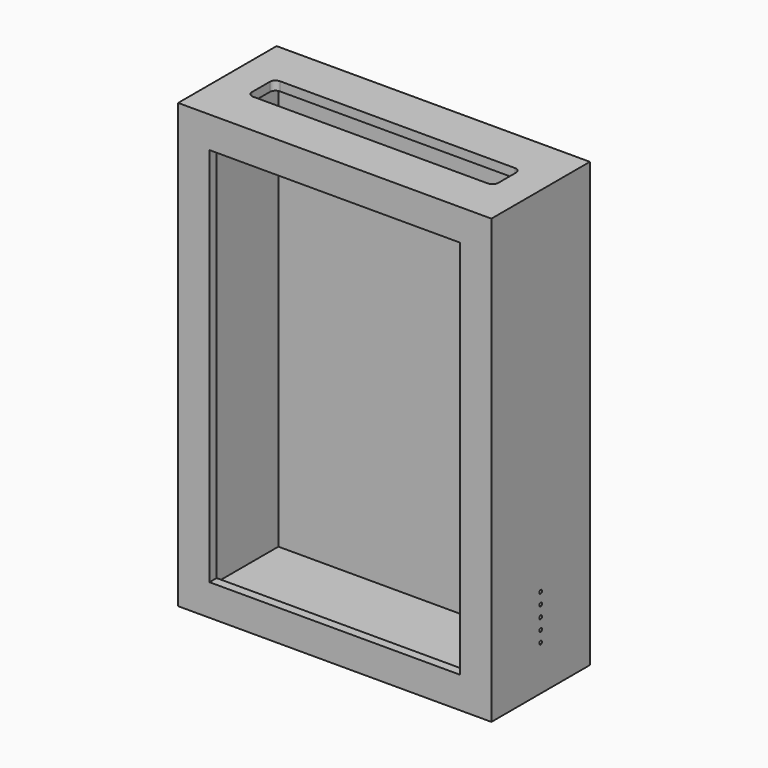
from build123d import *

# Parameters (mm, degrees)
F0_W      = 280
F0_H      = 110
F1_DEPTH  = 8
F2_W      = 280
F2_H      = 110
F2_W_2    = 264
F2_H_2    = 94
F3_DEPTH  = 20
F5_DEPTH  = 340
F7_DEPTH  = 20
F8_W      = 280
F8_H      = 110
F8_W_2    = 264
F8_H_2    = 94
F9_DEPTH  = 8
F10_R     = 1.55
F11_DEPTH = 8
F12_W     = 220
F12_H     = 30
F13_DEPTH = 8
F14_R     = 5


# Not quite as in the source:
# - a feature names something its author has since deleted; it is built from what else it names


with BuildPart() as f1:
    # F0 (on Top) → F1 (new body)
    with BuildSketch(Plane.XY):
        Rectangle(F0_W, F0_H)
    extrude(amount=F1_DEPTH)

    # F2 (on face) → F3 (join)
    with BuildSketch(Plane.XY.offset(8)):
        Rectangle(F2_W, F2_H)
        Rectangle(F2_W_2, F2_H_2, mode=Mode.SUBTRACT)
    extrude(amount=F3_DEPTH)

    # F4 (on face) → F5 (join)
    with BuildSketch(Plane.XY.offset(28)):
        Polygon((-132, -47), (-132, 47), (132, 47), (132, -47), (112, -47), (112, -55), (140, -55), (140, 55), (-140, 55), (-140, -55), (-112, -55), (-112, -47), align=None)
    extrude(amount=F5_DEPTH)

    # F6 (on face) → F7 (join)
    with BuildSketch(Plane.XY.offset(368)):
        Polygon((-140, -55), (-112, -55), (140, -55), (140, 55), (-140, 55), align=None)
        Polygon((-112, -47), (-132, -47), (-132, 47), (132, 47), (132, -47), align=None, mode=Mode.SUBTRACT)
    extrude(amount=F7_DEPTH)

    # F8 (on face) → F9 (join)
    with BuildSketch(Plane.XY.offset(388)):
        Rectangle(F8_W, F8_H)
        Rectangle(F8_W_2, F8_H_2, mode=Mode.SUBTRACT)
        Rectangle(F8_W_2, F8_H_2)
    extrude(amount=F9_DEPTH)

    # F10 (on face) → F11 (cut, through all)
    with BuildSketch(Plane.YZ.offset(140)):
        with Locations((0, 80)):
            Circle(F10_R)
        with Locations((0, 70)):
            Circle(F10_R)
        with Locations((0, 50)):
            Circle(F10_R)
        with Locations((0, 40)):
            Circle(F10_R)
        with Locations((0, 60)):
            Circle(F10_R)
    extrude(amount=-F11_DEPTH, mode=Mode.SUBTRACT)

    # F12 (on face) → F13 (cut, through all)
    with BuildSketch(Plane.XY.offset(396)):
        Rectangle(F12_W, F12_H)
    extrude(amount=-F13_DEPTH, mode=Mode.SUBTRACT)

    # F14
    f14_edges = [f1.edges().sort_by_distance(p)[0] for p in [
        (-110, 15, 392),
        (-110, -15, 392),
        (110, -15, 392),
        (110, 15, 392),
    ]]
    fillet(f14_edges, radius=F14_R)


solid = f1.part
